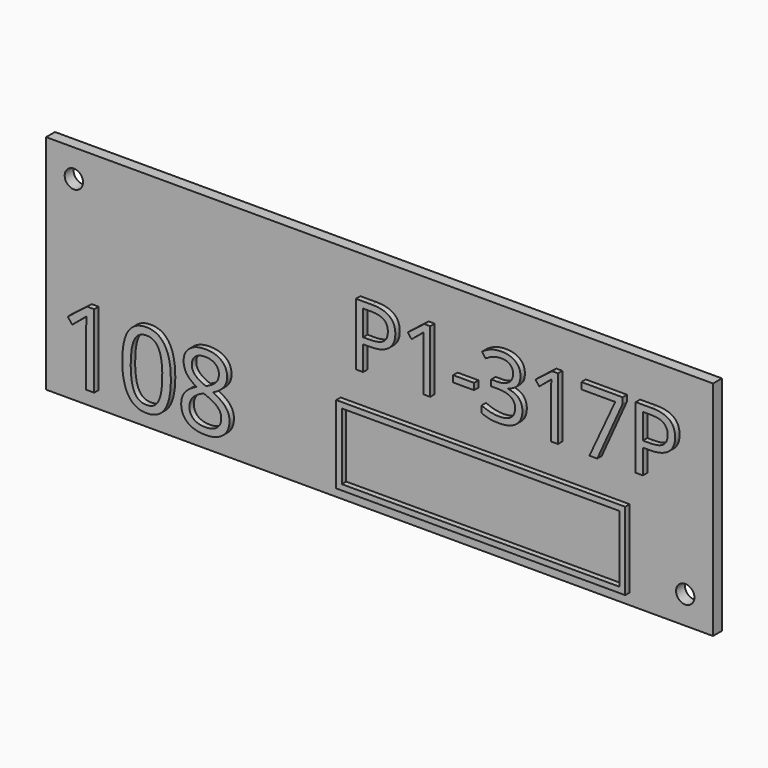
from build123d import *

# Parameters (mm, degrees)
F0_W         = 120
F0_H         = 40
F1_DEPTH     = 2
F3_D         = 3.3
F4_TEXT_SIZE = 15.681149951
F5_DEPTH     = 1
F6_TEXT_SIZE = 18.5155049272
F7_DEPTH     = 1
F8_W         = 52
F8_H         = 14
F8_W_2       = 49.99999962
F8_H_2       = 11.99999962
F9_DEPTH     = 1


# Not quite as in the source:
# - Text() gives the source's letters only with a copy of the font that has no kerning and outlines rounded to 1/6400 em; it was checked with that copy


with BuildPart() as f1:
    # F0 (on Front) → F1 (new body)
    with BuildSketch(Plane.XZ):
        Rectangle(F0_W, F0_H)
    extrude(amount=F1_DEPTH)

    # F3 (through all)
    with Locations(Plane.XZ.offset(2)):
        with Locations((-55, 15), (55, -15)):
            Hole(F3_D / 2)

    # F4 (on face) → F5 (join)
    with BuildSketch(Plane.XZ.offset(2)):
        with Locations((-5, 2)):
            Text('P1-317P', F4_TEXT_SIZE, font='Open Sans', text_align=(TextAlign.LEFT, TextAlign.BOTTOM))
    extrude(amount=F5_DEPTH)

    # F6 (on face) → F7 (join)
    with BuildSketch(Plane.XZ.offset(2)):
        with Locations((-57, -17)):
            Text('108', F6_TEXT_SIZE, font='Open Sans', text_align=(TextAlign.LEFT, TextAlign.BOTTOM))
    extrude(amount=F7_DEPTH)

    # F8 (on face) → F9 (join)
    with BuildSketch(Plane.XZ.offset(2)):
        with Locations((19, -11)):
            Rectangle(F8_W, F8_H)
        with Locations((19, -11)):
            Rectangle(F8_W_2, F8_H_2, mode=Mode.SUBTRACT)
    extrude(amount=F9_DEPTH)


solid = f1.part
